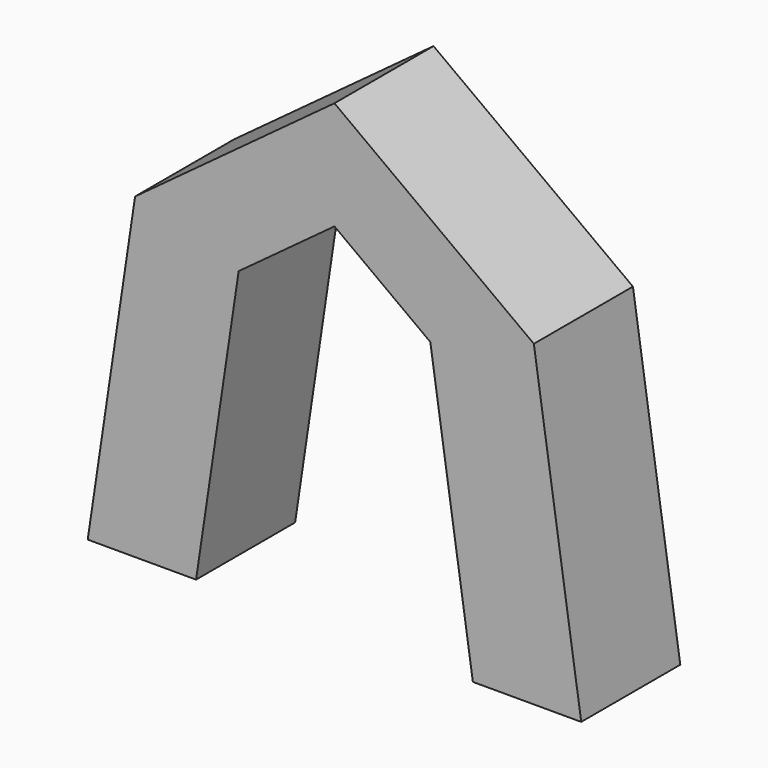
from build123d import *

# Parameters (mm, degrees)
F2_DEPTH = 4


# Not quite as in the source:
# - the program builds the solid bodies; features that only make, move or delete a surface that nothing else refers to are left out


with BuildPart() as f2:
    # F0 (on Front) → F2 (new body, symmetric)
    with BuildSketch(Plane.XZ):
        Polygon((-12.8808012232, 34.1780185699), (-15.9405209124, 13.6672500521), (-8.9405209124, 13.6672500521), (-6.189699587, 32.1073246897), (0, 36.6672500521), (6.189699587, 32.1073246897), (8.9405209124, 13.6672500521), (15.9405209124, 13.6672500521), (12.8808012232, 34.1780185699), (0, 43.6672500521), align=None)
    extrude(amount=F2_DEPTH, both=True)


solid = f2.part
